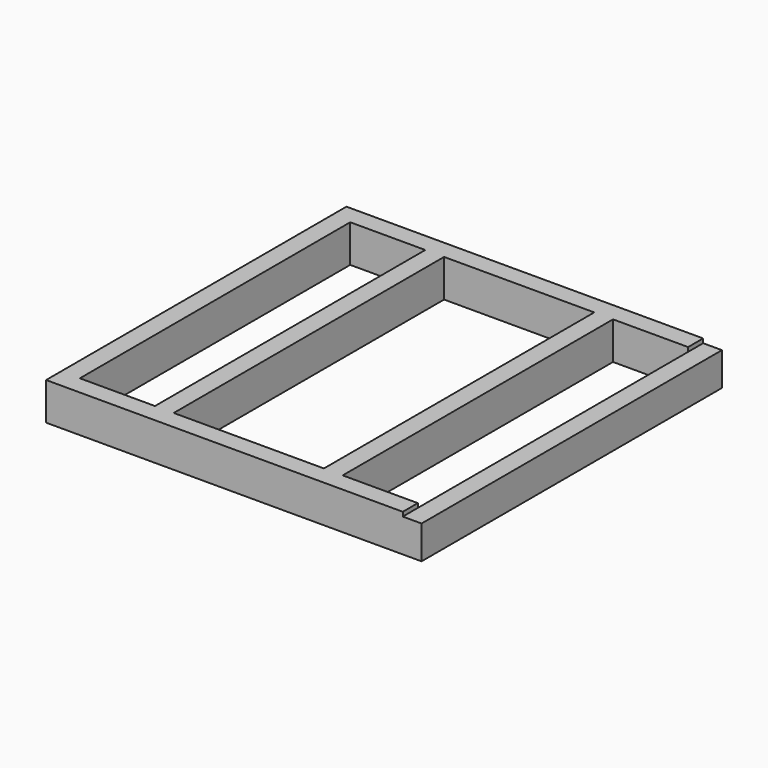
from build123d import *

# Parameters (mm, degrees)
F0_W        = 101.6
F0_H        = 457.1899072886
F0_W_2      = 203.2
F0_H_2      = 25.4
F1_DEPTH    = 50.8
F2_T        = 45.085
F2_T3_DEPTH = 140.97


# Not quite as in the source:
# - a shell that OpenCascade refuses in one call is made with other operations: the cavity is built on its own and cut out


with BuildPart() as f1:
    # F0 (on Top) → F1 (new body)
    with BuildSketch(Plane.XY):
        Polygon((-228.6, 213.5899730921), (-254, 213.5899730921), (-254, 188.1798803806), (-254, -213.5899730921), (-254, -294.4100269079), (-228.6, -294.4100269079), (-127, -294.4100269079), (-101.6, -294.4100269079), (-101.6, -269.0100269079), (-101.6, 188.1798803806), (-101.6, 188.1899730921), (101.6, 188.1899730921), (101.6, -269.0100269079), (101.6, -294.4100269079), (254, -294.4100269079), (254, -269.0100269079), (254, 213.5899730921), (101.6, 213.5899730921), (-101.6, 213.5899730921), (-127, 213.5899730921), align=None)
        with Locations((-177.8, -40.4150732636)):
            Rectangle(F0_W, F0_H, mode=Mode.SUBTRACT)
        with Locations((177.8, -40.4150732636)):
            Rectangle(F0_W, F0_H, mode=Mode.SUBTRACT)
        with Locations((0, -281.7100269079)):
            Rectangle(F0_W_2, F0_H_2)
    extrude(amount=F1_DEPTH)

    # F2: shell of thickness 45.085, made by hand


with BuildPart() as f2_core1:
    # F2_t2: copy of F1
    add(f1.part)

    # the walls: a layer under each face that stays
    f2_faces = [f2_core1.faces().sort_by_distance(p)[0] for p in [
        (-101.6, -40.4100269079, 25.4),
        (0, 188.1899730921, 25.4),
        (0, -269.0100269079, 25.4),
        (-228.6, -40.4150732636, 25.4),
        (-177.8, 188.1798803806, 25.4),
        (-177.8, -269.0100269079, 25.4),
        (177.8, 188.1798803806, 25.4),
        (177.8, -269.0100269079, 25.4),
        (127, -40.4150732636, 25.4),
        (-237.0666666667, -277.4766935746, 0),
    ]]
    thicken(f2_faces, amount=-F2_T, mode=Mode.SUBTRACT)

    # F2_s4 → F2_t3 (cut)
    with BuildSketch(Plane.XY.offset(-45.085)):
        Polygon((-101.14915, -268.5591769079), (-146.685, -269.0100269079), (-146.685, -314.0950269079), (-101.6, -314.0950269079), align=None)
        Polygon((-101.14915, 187.7391230921), (-146.685, 188.1899730921), (-146.685, 233.2749730921), (-101.6, 233.2749730921), align=None)
        Polygon((-228.14915, -268.5591769079), (-273.685, -269.0100269079), (-273.685, -314.0950269079), (-228.6, -314.0950269079), align=None)
        Polygon((-228.14915, 187.7290303806), (-273.685, 188.1798803806), (-273.685, 233.2648803806), (-228.6, 233.2648803806), align=None)
        Polygon((127.45085, 187.7290303806), (127, 233.2648803806), (81.915, 233.2648803806), (81.915, 188.1798803806), align=None)
        Polygon((127.45085, -268.5591769079), (127, -314.0950269079), (81.915, -314.0950269079), (81.915, -269.0100269079), align=None)
    extrude(amount=F2_T3_DEPTH, mode=Mode.SUBTRACT)


with BuildPart() as f1_1:
    add(f1.part)

    # what is left inside the walls is the cavity
    f2_cavity = [f2_core1.part.solids().sort_by_distance(p)[0] for p in [
        (241.3, -125.076694, 45.53585),
    ]]
    add(f2_cavity, mode=Mode.SUBTRACT)


solid = f1_1.part
